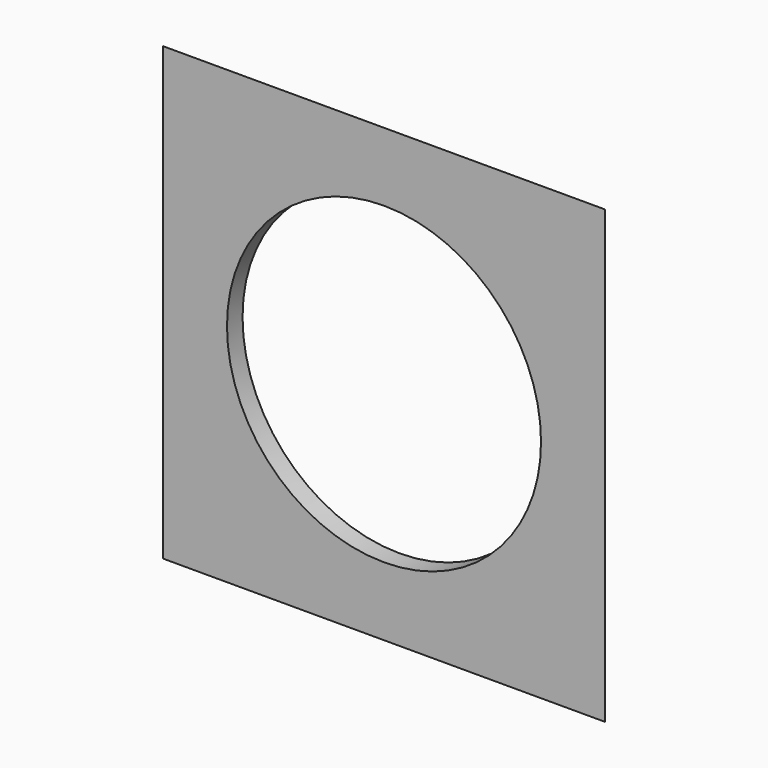
from build123d import *

# Parameters (mm, degrees)
F0_W     = 500
F0_H     = 510
F0_R     = 177.5
F1_DEPTH = 22
F2_SIZE  = 21.99999


# Not quite as in the source:
# - a fillet or chamfer is up to 0.001 mm smaller than in the source, because OpenCascade refuses the exact size


with BuildPart() as f1:
    # F0 (on Front) → F1 (new body)
    with BuildSketch(Plane.XZ):
        Rectangle(F0_W, F0_H)
        with BuildLine():
            Line((-161.5, 206.5), (161.5, 206.5))
            ThreePointArc((161.5, 206.5), (189.7842712475, 194.7842712475), (201.5, 166.5))
            Line((201.5, 166.5), (201.5, -166.5))
            ThreePointArc((201.5, -166.5), (189.7842712475, -194.7842712475), (161.5, -206.5))
            Line((161.5, -206.5), (-161.5, -206.5))
            ThreePointArc((-161.5, -206.5), (-189.7842712475, -194.7842712475), (-201.5, -166.5))
            Line((-201.5, -166.5), (-201.5, 166.5))
            ThreePointArc((-201.5, 166.5), (-189.7842712475, 194.7842712475), (-161.5, 206.5))
        make_face(mode=Mode.SUBTRACT)
        with BuildLine():
            ThreePointArc((201.5, 166.5), (189.7842712475, 194.7842712475), (161.5, 206.5))
            Line((161.5, 206.5), (-161.5, 206.5))
            ThreePointArc((-161.5, 206.5), (-189.7842712475, 194.7842712475), (-201.5, 166.5))
            Line((-201.5, 166.5), (-201.5, -166.5))
            ThreePointArc((-201.5, -166.5), (-189.7842712475, -194.7842712475), (-161.5, -206.5))
            Line((-161.5, -206.5), (161.5, -206.5))
            ThreePointArc((161.5, -206.5), (189.7842712475, -194.7842712475), (201.5, -166.5))
            Line((201.5, -166.5), (201.5, 166.5))
        make_face()
        Circle(F0_R, mode=Mode.SUBTRACT)
    extrude(amount=F1_DEPTH)

    # F2 (size 22 in the source; OpenCascade refuses exactly that, so slightly less here)
    f2_edges = [f1.edges().sort_by_distance(p)[0] for p in [
        (0, 0, 255),
        (250, 0, 0),
        (0, 0, -255),
        (-250, 0, 0),
    ]]
    chamfer(f2_edges, length=F2_SIZE)


solid = f1.part
